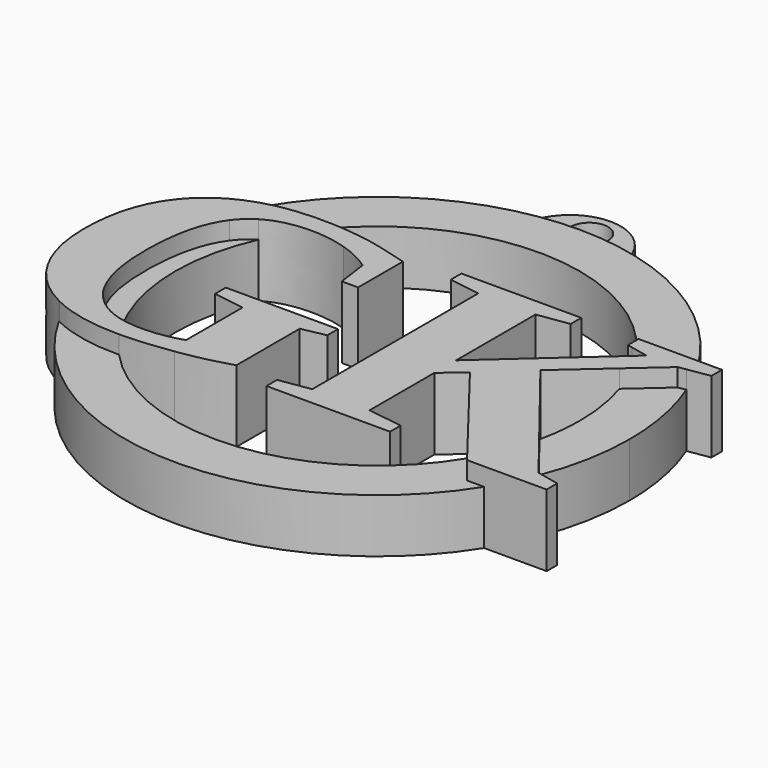
from build123d import *

# Parameters (mm, degrees)
F1_DEPTH = 6.096
F2_DEPTH = 4.572
F0_R     = 1.5875
F3_DEPTH = 3.175


with BuildPart() as f1:
    # F0 (on Top) → F1 (new body)
    with BuildSketch(Plane.XY):
        with BuildLine():
            Line((13.1990751617, 4.6464640634), (17.129461098, 8.1167903742))
            ThreePointArc((17.129461098, 8.1167903742), (16.8217445929, 8.9971059692), (16.4666606544, 9.8594054479))
            Line((16.4666606544, 9.8594054479), (7.9593701355, 2.2607470054))
            Line((7.9593701355, 2.2607470054), (7.9593701355, 10.6699067182))
            Line((7.9593701355, 10.6699067182), (10.6260497396, 11.0740984512))
            Line((10.6260497396, 11.0740984512), (10.6260497396, 12.1979486355))
            Line((10.6260497396, 12.1979486355), (0.4571772382, 12.1979486355))
            Line((0.4571772382, 12.1979486355), (0.4571772382, 11.0740984512))
            Line((0.4571772382, 11.0740984512), (3.1090693399, 10.6699067182))
            Line((3.1090693399, 10.6699067182), (3.1090693399, -6.9173628335))
            Line((3.1090693399, -6.9173628335), (0.4571772382, -7.3363420689))
            Line((0.4571772382, -7.3363420689), (0.4571772382, -8.4601922533))
            Line((0.4571772382, -8.4601922533), (10.9316581231, -8.4601922533))
            Line((10.9316581231, -8.4601922533), (10.9316581231, -7.3363420689))
            Line((10.9316581231, -7.3363420689), (7.9593701355, -6.9173628335))
            Line((7.9593701355, -6.9173628335), (7.9593701355, -0.0510325405))
            Line((7.9593701355, -0.0510325405), (9.748657929, 1.4917968793))
            Line((9.748657929, 1.4917968793), (15.4999066991, -5.927865272))
            ThreePointArc((15.4999066991, -5.927865272), (16.7161227426, -3.4746609665), (17.5266633254, -0.8592419192))
            Line((17.5266633254, -0.8592419192), (13.1990751617, 4.6464640634))
        make_face()
        with BuildLine():
            ThreePointArc((16.4666606544, 9.8594054479), (16.8217445929, 8.9971059692), (17.129461098, 8.1167903742))
            Line((17.129461098, 8.1167903742), (20.0210429475, 10.6699067182))
            Line((20.0210429475, 10.6699067182), (20.6703936904, 10.7737015738))
            ThreePointArc((20.6703936904, 10.7737015738), (20.3708801374, 11.4915066696), (20.0454692082, 12.1979486355))
            Line((20.0454692082, 12.1979486355), (15.4763505353, 12.1979486355))
            Line((15.4763505353, 12.1979486355), (15.4763505353, 11.7602529477))
            ThreePointArc((15.4763505353, 11.7602529477), (15.7031816224, 11.3728515682), (15.9198012697, 10.9796492038))
            Line((15.9198012697, 10.9796492038), (17.3740800133, 10.6699067182))
            Line((17.3740800133, 10.6699067182), (16.4666606544, 9.8594054479))
        make_face()
        with BuildLine():
            ThreePointArc((20.0454692082, 12.1979486355), (20.3708801374, 11.4915066696), (20.6703936904, 10.7737015738))
            Line((20.6703936904, 10.7737015738), (22.5497058623, 11.0740984512))
            Line((22.5497058623, 11.0740984512), (22.5497058623, 12.1979486355))
            Line((22.5497058623, 12.1979486355), (20.0454692082, 12.1979486355))
        make_face()
        with BuildLine():
            Line((20.7023127689, -4.8994119814), (17.5266633254, -0.8592419192))
            ThreePointArc((17.5266633254, -0.8592419192), (16.7161227426, -3.4746609665), (15.4999066991, -5.927865272))
            Line((15.4999066991, -5.927865272), (17.4628050278, -8.4601922533))
            Line((17.4628050278, -8.4601922533), (18.9098256888, -8.4601922533))
            ThreePointArc((18.9098256888, -8.4601922533), (19.8891997575, -6.7216497988), (20.7023127689, -4.8994119814))
        make_face()
        with BuildLine():
            Line((22.2884599861, -6.9173628335), (20.7023127689, -4.8994119814))
            ThreePointArc((20.7023127689, -4.8994119814), (19.8891997575, -6.7216497988), (18.9098256888, -8.4601922533))
            Line((18.9098256888, -8.4601922533), (24.2108353014, -8.4601922533))
            Line((24.2108353014, -8.4601922533), (24.2108353014, -7.3363420689))
            Line((24.2108353014, -7.3363420689), (22.2884599861, -6.9173628335))
        make_face()
        with BuildLine():
            Line((15.4763505353, 11.0740984512), (15.9198012697, 10.9796492038))
            ThreePointArc((15.9198012697, 10.9796492038), (15.7031816224, 11.3728515682), (15.4763505353, 11.7602529477))
            Line((15.4763505353, 11.7602529477), (15.4763505353, 11.0740984512))
        make_face()
    extrude(amount=F1_DEPTH)



with BuildPart() as f1b:
    # F0 (on Top) → F1, piece 2 (new body)
    with BuildSketch(Plane.XY):
        with BuildLine():
            add(Edge.make_bspline(
                [(-13.5465420725, 12.3386346598), (-12.6387551901, 12.4296195068), (-11.6488580811, 12.4296195068)],
                knots=[0.819888429, 0.819888429, 0.819888429, 1, 1, 1], degree=2))
            ThreePointArc((-13.5465420725, 12.3386346598), (-14.2660777227, 11.1436447733), (-14.8861798945, 9.8941626097))
            add(Edge.make_bspline(
                [(-11.0918621563, 10.8079234075), (-13.3874045962, 10.8079234075), (-14.8861798945, 9.8941626097)],
                knots=[0, 0, 0, 0.6397059246, 0.6397059246, 0.6397059246], degree=2))
            add(Edge.make_bspline(
                [(-8.0752116615, 10.3470462486), (-9.5391744016, 10.8079234075), (-11.0918621563, 10.8079234075)],
                knots=[0, 0, 0, 1, 1, 1], degree=2))
            add(Edge.make_bspline(
                [(-5.393744555, 9.0531397863), (-6.6112489213, 9.8861690896), (-8.0752116615, 10.3470462486)],
                knots=[0, 0, 0, 1, 1, 1], degree=2))
            Line((-5.393744555, 9.0531397863), (-5.0240569943, 6.3716726798))
            Line((-5.0240569943, 6.3716726798), (-3.6389609338, 6.3716726798))
            Line((-3.6389609338, 6.3716726798), (-3.6389609338, 11.1184609584))
            add(Edge.make_bspline(
                [(-7.1485281761, 12.0278923576), (-6.1922696859, 11.8430485773), (-3.6389609338, 11.1184609584)],
                knots=[0, 0, 0, 1, 1, 1], degree=2))
            add(Edge.make_bspline(
                [(-9.2064555971, 12.3211778224), (-8.1047866663, 12.2127361379), (-7.1485281761, 12.0278923576)],
                knots=[0, 0, 0, 1, 1, 1], degree=2))
            add(Edge.make_bspline(
                [(-11.6488580811, 12.4296195068), (-10.3081245278, 12.4296195068), (-9.2064555971, 12.3211778224)],
                knots=[0, 0, 0, 1, 1, 1], degree=2))
        make_face()
        with BuildLine():
            ThreePointArc((-13.2947500331, -6.9168666563), (-12.5802923039, -7.8694978593), (-11.801489684, -8.7702878097))
            add(Edge.make_bspline(
                [(-7.3974511336, -8.3911839086), (-9.8374422228, -8.7577776918), (-11.801489684, -8.7702878097)],
                knots=[0, 0, 0, 0.9658747135, 0.9658747135, 0.9658747135], degree=2))
            add(Edge.make_bspline(
                [(-2.9587358222, -7.3807045762), (-4.8712528026, -8.011638013), (-7.3974511336, -8.3911839086)],
                knots=[0, 0, 0, 1, 1, 1], degree=2))
            Line((-2.9587358222, -7.3807045762), (-2.9587358222, -0.6671784749))
            Line((-2.9587358222, -0.6671784749), (-0.9427063248, -0.2629867419))
            Line((-0.9427063248, -0.2629867419), (-0.9427063248, 0.8756509448))
            Line((-0.9427063248, 0.8756509448), (-10.4609287195, 0.8756509448))
            Line((-10.4609287195, 0.8756509448), (-10.4609287195, -0.2629867419))
            Line((-10.4609287195, -0.2629867419), (-7.8139657853, -0.6671784749))
            Line((-7.8139657853, -0.6671784749), (-7.8139657853, -6.6413294549))
            add(Edge.make_bspline(
                [(-11.2150913432, -7.1835378772), (-9.4307327172, -7.1835378772), (-7.8139657853, -6.6413294549)],
                knots=[0, 0, 0, 1, 1, 1], degree=2))
            add(Edge.make_bspline(
                [(-13.2947500331, -6.9168666563), (-12.3470834343, -7.1835378772), (-11.2150913432, -7.1835378772)],
                knots=[0.6551775055, 0.6551775055, 0.6551775055, 1, 1, 1], degree=2))
        make_face()
        with BuildLine():
            add(Edge.make_bspline(
                [(-11.801489684, -8.7702878097), (-11.8708813778, -8.7707298042), (-11.9396789621, -8.7707298042)],
                knots=[0.9658747135, 0.9658747135, 0.9658747135, 1, 1, 1], degree=2))
            ThreePointArc((-11.801489684, -8.7702878097), (-12.5802923039, -7.8694978593), (-13.2947500331, -6.9168666563))
            add(Edge.make_bspline(
                [(-16.2305192493, -4.940766676), (-15.095357152, -6.4101799171), (-13.2947500331, -6.9168666563)],
                knots=[0, 0, 0, 0.6551775055, 0.6551775055, 0.6551775055], degree=2))
            add(Edge.make_bspline(
                [(-17.9631216169, 1.6593885734), (-17.9631216169, -2.6979954747), (-16.2305192493, -4.940766676)],
                knots=[0, 0, 0, 1, 1, 1], degree=2))
            add(Edge.make_bspline(
                [(-16.3217088476, 8.5750105412), (-17.9631216169, 6.3420976749), (-17.9631216169, 1.6593885734)],
                knots=[0, 0, 0, 1, 1, 1], degree=2))
            add(Edge.make_bspline(
                [(-14.8861798945, 9.8941626097), (-15.7303175515, 9.3795158179), (-16.3217088476, 8.5750105412)],
                knots=[0.6397059246, 0.6397059246, 0.6397059246, 1, 1, 1], degree=2))
            ThreePointArc((-14.8861798945, 9.8941626097), (-14.2660777227, 11.1436447733), (-13.5465420725, 12.3386346598))
            add(Edge.make_bspline(
                [(-19.2795180694, 10.3190176516), (-17.0109804199, 11.9914040496), (-13.5465420725, 12.3386346598)],
                knots=[0.1325184685, 0.1325184685, 0.1325184685, 0.819888429, 0.819888429, 0.819888429], degree=2))
            ThreePointArc((-19.2795180694, 10.3190176516), (-20.5461171043, 1.2635766126), (-17.9156975267, -7.4934878711))
            add(Edge.make_bspline(
                [(-17.830034095, -7.5359733517), (-17.8730342479, -7.5148940204), (-17.9156975267, -7.4934878711)],
                knots=[0, 0, 0, 0.017071651, 0.017071651, 0.017071651], degree=2))
            add(Edge.make_bspline(
                [(-11.9396789621, -8.7707298042), (-15.3112295152, -8.7707298042), (-17.830034095, -7.5359733517)],
                knots=[0, 0, 0, 1, 1, 1], degree=2))
        make_face()
        with BuildLine():
            add(Edge.make_bspline(
                [(-17.9156975267, -7.4934878711), (-20.3721058809, -6.2609936642), (-21.7117534818, -3.945074846)],
                knots=[0.017071651, 0.017071651, 0.017071651, 1, 1, 1], degree=2))
            ThreePointArc((-17.9156975267, -7.4934878711), (-20.5461171043, 1.2635766126), (-19.2795180694, 10.3190176516))
            add(Edge.make_bspline(
                [(-20.1097740523, 9.6249232134), (-19.7168708088, 9.9965972709), (-19.2795180694, 10.3190176516)],
                knots=[0, 0, 0, 0.1325184685, 0.1325184685, 0.1325184685], degree=2))
            add(Edge.make_bspline(
                [(-23.0746682887, 1.6298135686), (-23.0746682887, 6.82022692), (-20.1097740523, 9.6249232134)],
                knots=[0, 0, 0, 1, 1, 1], degree=2))
            add(Edge.make_bspline(
                [(-21.7117534818, -3.945074846), (-23.0746682887, -1.5889327928), (-23.0746682887, 1.6298135686)],
                knots=[0, 0, 0, 1, 1, 1], degree=2))
        make_face()
    extrude(amount=F1_DEPTH)


with BuildPart() as f1_1:
    add(f1.part)

    add(f1b.part)  # F2 merges F1b
    # F0 (on Top) → F2 (join)
    with BuildSketch(Plane.XY):
        with BuildLine():
            ThreePointArc((-13.5465420725, 12.3386346598), (1.1244113714, 20.0534288841), (15.4763505353, 11.7602529477))
            Line((15.4763505353, 11.7602529477), (15.4763505353, 12.1979486355))
            Line((15.4763505353, 12.1979486355), (20.0454692082, 12.1979486355))
            ThreePointArc((20.0454692082, 12.1979486355), (13.6054197321, 20.0182214035), (4.2892900104, 23.9982503516))
            ThreePointArc((4.2892900104, 23.9982503516), (0, 24.2733374292), (-4.2576981592, 23.685384983))
            ThreePointArc((-4.2576981592, 23.685384983), (-13.4370376563, 18.8772693512), (-19.2795180694, 10.3190176516))
            add(Edge.make_bspline(
                [(-19.2795180694, 10.3190176516), (-17.0109804199, 11.9914040496), (-13.5465420725, 12.3386346598)],
                knots=[0.1325184685, 0.1325184685, 0.1325184685, 0.819888429, 0.819888429, 0.819888429], degree=2))
        make_face()
        with BuildLine():
            add(Edge.make_bspline(
                [(-16.2305192493, -4.940766676), (-15.095357152, -6.4101799171), (-13.2947500331, -6.9168666563)],
                knots=[0, 0, 0, 0.6551775055, 0.6551775055, 0.6551775055], degree=2))
            ThreePointArc((-13.2947500331, -6.9168666563), (-16.3013447934, 1.2793532259), (-14.8861798945, 9.8941626097))
            add(Edge.make_bspline(
                [(-14.8861798945, 9.8941626097), (-15.7303175515, 9.3795158179), (-16.3217088476, 8.5750105412)],
                knots=[0.6397059246, 0.6397059246, 0.6397059246, 1, 1, 1], degree=2))
            add(Edge.make_bspline(
                [(-16.3217088476, 8.5750105412), (-17.9631216169, 6.3420976749), (-17.9631216169, 1.6593885734)],
                knots=[0, 0, 0, 1, 1, 1], degree=2))
            add(Edge.make_bspline(
                [(-17.9631216169, 1.6593885734), (-17.9631216169, -2.6979954747), (-16.2305192493, -4.940766676)],
                knots=[0, 0, 0, 1, 1, 1], degree=2))
        make_face()
        with BuildLine():
            Line((17.4628050278, -8.4601922533), (15.4999066991, -5.927865272))
            ThreePointArc((15.4999066991, -5.927865272), (2.5594951508, -14.1713617347), (-11.801489684, -8.7702878097))
            add(Edge.make_bspline(
                [(-11.801489684, -8.7702878097), (-11.8708813778, -8.7707298042), (-11.9396789621, -8.7707298042)],
                knots=[0.9658747135, 0.9658747135, 0.9658747135, 1, 1, 1], degree=2))
            add(Edge.make_bspline(
                [(-11.9396789621, -8.7707298042), (-15.3112295152, -8.7707298042), (-17.830034095, -7.5359733517)],
                knots=[0, 0, 0, 1, 1, 1], degree=2))
            add(Edge.make_bspline(
                [(-17.830034095, -7.5359733517), (-17.8730342479, -7.5148940204), (-17.9156975267, -7.4934878711)],
                knots=[0, 0, 0, 0.017071651, 0.017071651, 0.017071651], degree=2))
            ThreePointArc((-17.9156975267, -7.4934878711), (0.2211607621, -18.4870686939), (18.9098256888, -8.4601922533))
            Line((18.9098256888, -8.4601922533), (17.4628050278, -8.4601922533))
        make_face()
        with BuildLine():
            ThreePointArc((17.129461098, 8.1167903742), (17.7381923934, 5.5381853901), (17.9427280894, 2.8966096097))
            ThreePointArc((17.9427280894, 2.8966096097), (17.8383947275, 1.0071963016), (17.5266633254, -0.8592419192))
            Line((17.5266633254, -0.8592419192), (20.7023127689, -4.8994119814))
            ThreePointArc((20.7023127689, -4.8994119814), (21.8025208752, -1.0702053402), (22.173547196, 2.8966096097))
            ThreePointArc((22.173547196, 2.8966096097), (21.7943986847, 6.9062245623), (20.6703936904, 10.7737015738))
            Line((20.6703936904, 10.7737015738), (20.0210429475, 10.6699067182))
            Line((20.0210429475, 10.6699067182), (17.129461098, 8.1167903742))
        make_face()
        with BuildLine():
            ThreePointArc((15.9198012697, 10.9796492038), (16.2034067616, 10.424494755), (16.4666606544, 9.8594054479))
            Line((16.4666606544, 9.8594054479), (17.3740800133, 10.6699067182))
            Line((17.3740800133, 10.6699067182), (15.9198012697, 10.9796492038))
        make_face()
    extrude(amount=F2_DEPTH)

    # F0 (on Top) → F3 (join)
    with BuildSketch(Plane.XY):
        with BuildLine():
            ThreePointArc((-4.2576981592, 23.685384983), (0, 24.2733374292), (4.2892900104, 23.9982503516))
            ThreePointArc((4.2892900104, 23.9982503516), (-0.1572281654, 28.5685628013), (-4.2576981592, 23.685384983))
        make_face()
        with Locations((0, 26.3267960399)):
            Circle(F0_R, mode=Mode.SUBTRACT)
    extrude(amount=F3_DEPTH)


solid = f1_1.part
